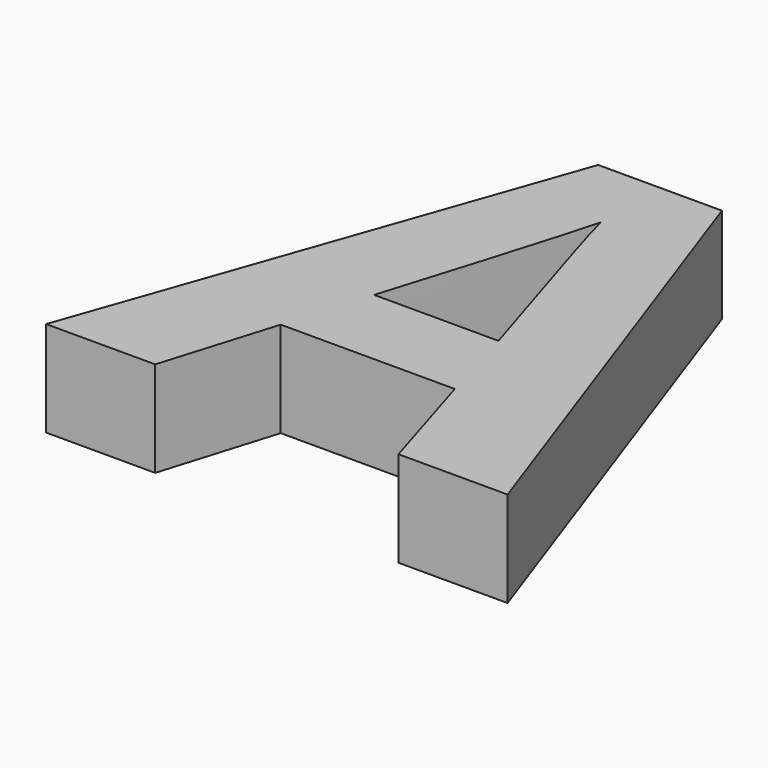
from build123d import *

# Parameters (mm, degrees)
F0_TEXT_SIZE = 44.4499995663
F1_DEPTH     = 6.35


# Not quite as in the source:
# - Text() gives the source's letters only with a copy of the font that has no kerning and outlines rounded to 1/6400 em; it was checked with that copy


with BuildPart() as f1:
    # F0 (on Top) → F1 (new body)
    with BuildSketch(Plane.XY):
        with Locations((-18.8641455024, -8.5864393041)):
            Text('A', F0_TEXT_SIZE, font='Open Sans', font_style=FontStyle.BOLD, text_align=(TextAlign.LEFT, TextAlign.BOTTOM))
    extrude(amount=F1_DEPTH)


solid = f1.part
